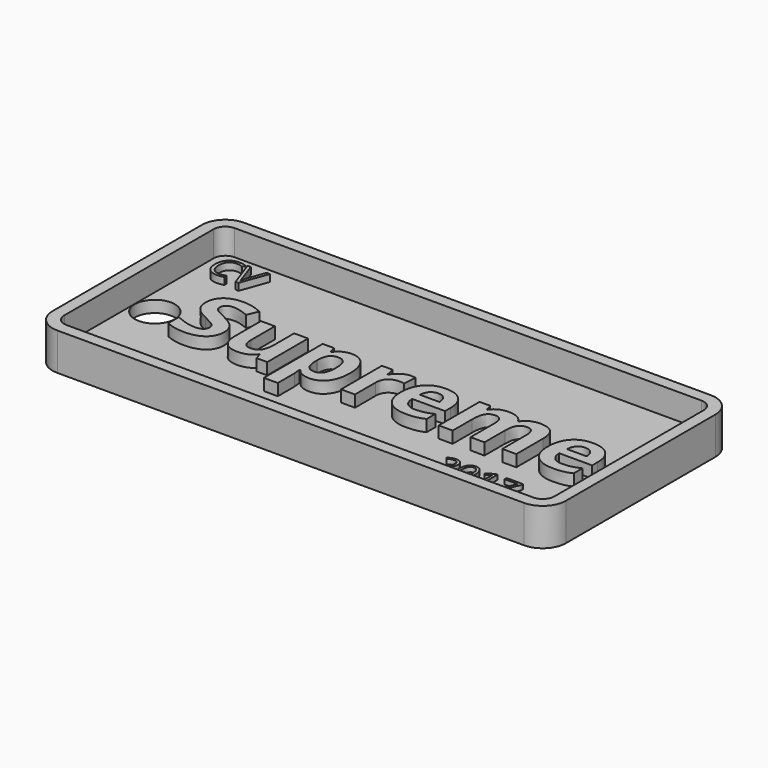
from build123d import *

# Parameters (mm, degrees)
F0_W          = 110
F0_H          = 50
F1_DEPTH      = 8
F2_R          = 5
F3_T          = -2.5
F5_R          = 4.3038983247
F6_DEPTH      = 25
F7_TEXT_SIZE  = 20.0358749781
F8_DEPTH      = 2.5
F9_TEXT_SIZE  = 8.0746624412
F10_DEPTH     = 1.5
F11_TEXT_SIZE = 7.3406043359
F12_DEPTH     = 1


# Not quite as in the source:
# - Text() gives the source's letters only with a copy of the font that has no kerning and outlines rounded to 1/6400 em; it was checked with that copy


with BuildPart() as f1:
    # F0 (on Top) → F1 (new body)
    with BuildSketch(Plane.XY):
        with Locations((-9.8998378962, 1.2335861551)):
            Rectangle(F0_W, F0_H)
    extrude(amount=F1_DEPTH)

    # F2
    f2_edges = [f1.edges().sort_by_distance(p)[0] for p in [
        (45.100162, -23.766414, 4),
        (45.100162, 26.233586, 4),
        (-64.899838, 26.233586, 4),
        (-64.899838, -23.766414, 4),
    ]]
    fillet(f2_edges, radius=F2_R)

    # F3
    f3_openings = [f1.faces().sort_by_distance(p)[0] for p in [
        (-9.899838, 1.233586, 8),
    ]]
    offset(amount=F3_T, openings=f3_openings)

    # F5 (on face) → F6 (cut)
    with BuildSketch(Plane.XY.offset(2.5)):
        with Locations((-58.0054558814, 0)):
            Circle(F5_R)
    extrude(amount=-F6_DEPTH, mode=Mode.SUBTRACT)

    # F7 (on face) → F8 (join)
    with BuildSketch(Plane.XY.offset(2.5)):
        with Locations((-51.5535660088, -6.2664138449)):
            Text('Supreme', F7_TEXT_SIZE, font='Open Sans', font_style=FontStyle.BOLD, text_align=(TextAlign.LEFT, TextAlign.BOTTOM))
    extrude(amount=F8_DEPTH)

    # F9 (on face) → F10 (join)
    with BuildSketch(Plane.XY.offset(2.5)):
        with Locations((-59.5910251141, 14.6665275097)):
            Text('CV', F9_TEXT_SIZE, font='Open Sans', text_align=(TextAlign.LEFT, TextAlign.BOTTOM))
    extrude(amount=F10_DEPTH)

    # F11 (on face) → F12 (join)
    with BuildSketch(Plane.XY.offset(2.5)):
        with Locations((13.8737428933, -17.0448832214)):
            Text('2017', F11_TEXT_SIZE, font='Open Sans', text_align=(TextAlign.LEFT, TextAlign.BOTTOM))
    extrude(amount=F12_DEPTH)


solid = f1.part
